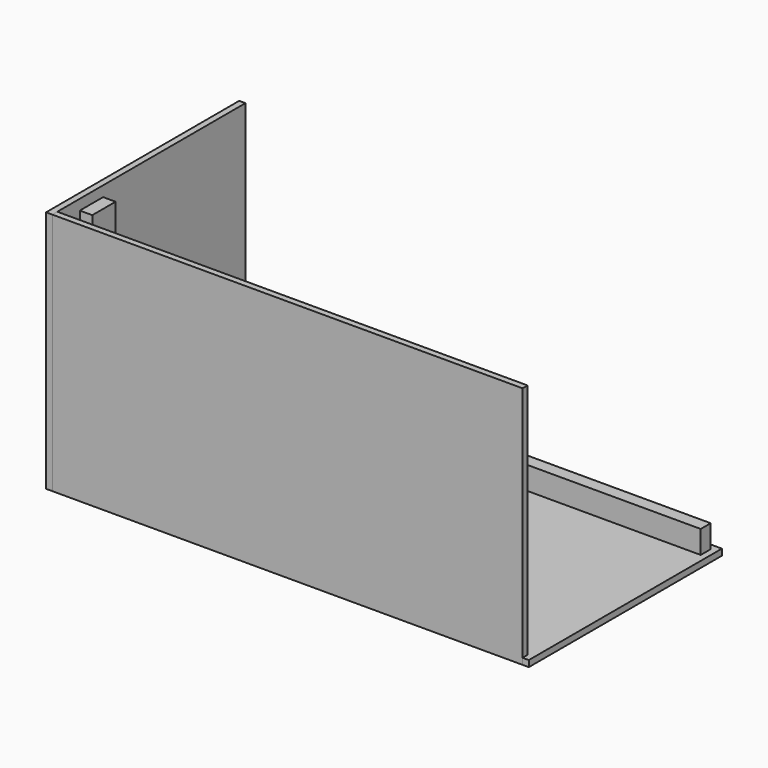
from build123d import *

# Parameters (mm, degrees)
F4_W      = 1473.2
F4_H      = 736.6
F7_DEPTH  = 19.05
F8_DEPTH  = 742.95
F5_W      = 1435.1
F5_H      = 19.05
F9_DEPTH  = 742.95
F10_DEPTH = 88.9
F5_W_2    = 38.1
F5_H_2    = 622.3
F11_DEPTH = 88.9
F6_W      = 38.1
F6_H      = 88.9
F12_DEPTH = 742.95


# Not quite as in the source:
# - a length typed as a fraction of an inch, garbled in the dataset ("3 / 203.2 mm" for 3/8 in), is restored


with BuildPart() as f7:
    # F4 (on Top) → F7 (new body)
    with BuildSketch(Plane.XY):
        Rectangle(F4_W, F4_H)
    extrude(amount=F7_DEPTH)


with BuildPart() as f8:
    # F5 (on Top) → F8 (new body)
    with BuildSketch(Plane.XY):
        Polygon((-717.55, 368.3), (-736.6, 368.3), (-736.6, -368.3), (-717.55, -368.3), (-717.55, -349.25), (-717.55, -311.15), (-717.55, 311.15), (-717.55, 349.25), align=None)
    extrude(amount=F8_DEPTH)


with BuildPart() as f9:
    # F5 (on Top) → F9 (new body)
    with BuildSketch(Plane.XY):
        with Locations((0, -358.775)):
            Rectangle(F5_W, F5_H)
    extrude(amount=F9_DEPTH)


with BuildPart() as f10:
    # F5 (on Top) → F10 (new body)
    with BuildSketch(Plane.XY):
        Polygon((717.55, 349.25), (-717.55, 349.25), (-717.55, 311.15), (-679.45, 311.15), (-57.15, 311.15), (-19.05, 311.15), (679.45, 311.15), (717.55, 311.15), align=None)
    extrude(amount=F10_DEPTH)


with BuildPart() as f11:
    # F5 (on Top) → F11 (new body)
    with BuildSketch(Plane.XY):
        with Locations((-698.5, 0)):
            Rectangle(F5_W_2, F5_H_2)
    extrude(amount=F11_DEPTH)


with BuildPart() as f12:
    # F6 (on Top) → F12 (new body)
    with BuildSketch(Plane.XY):
        with Locations((-660.4, -266.7)):
            Rectangle(F6_W, F6_H)
    extrude(amount=F12_DEPTH)


solid = Compound([f7.part, f8.part, f9.part, f10.part, f11.part, f12.part])
